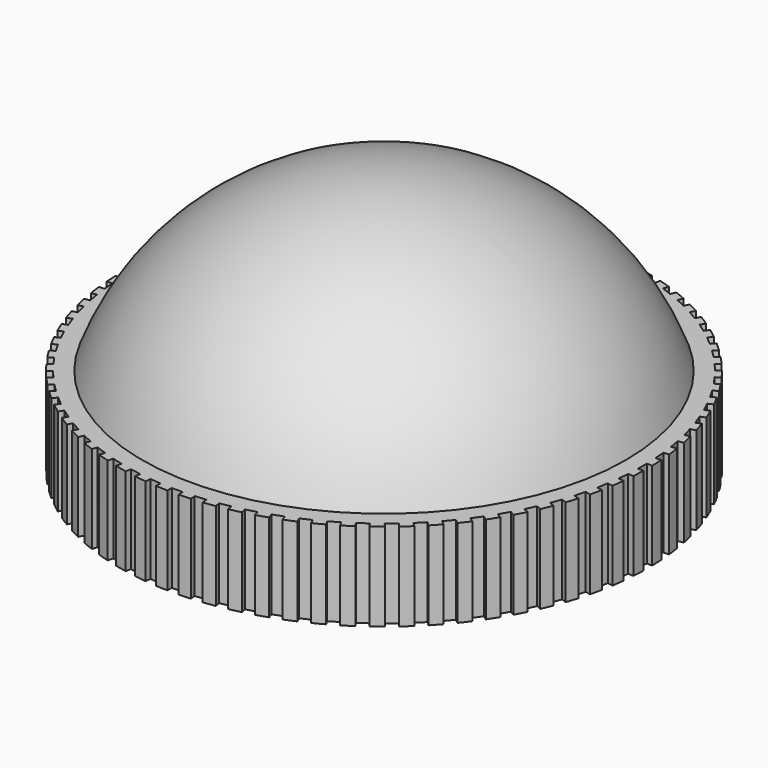
from build123d import *

# Parameters (mm, degrees)
F0_R            = 9.525
F0_R_2          = 6.35
F1_DEPTH        = 3.175
F5_DEPTH        = 25.4
F5_COPIES_COUNT = 72


# Not quite as in the source:
# - a pattern or mirror of a feature is missing from the dataset's text; its kind, count and spacing are read off the source's solid


with BuildPart() as f1:
    # F0 (on Top) → F1 (new body)
    with BuildSketch(Plane.XY):
        Circle(F0_R)
        Circle(F0_R_2, mode=Mode.SUBTRACT)
    extrude(amount=F1_DEPTH)

    # F4 (on face) → F5 (cut)
    with BuildSketch(Plane.XY.offset(3.175)):
        with BuildLine():
            Line((0.1984375, -9.5229327184), (0.1984375, -9.3265625))
            Line((0.1984375, -9.3265625), (-0.1984375, -9.3265625))
            Line((-0.1984375, -9.3265625), (-0.1984375, -9.5229327184))
            ThreePointArc((-0.1984375, -9.5229327184), (0, -9.525), (0.1984375, -9.5229327184))
        make_face()
        with BuildLine():
            Line((0.1984375, -9.7234375), (0.1984375, -9.5229327184))
            ThreePointArc((0.1984375, -9.5229327184), (0, -9.525), (-0.1984375, -9.5229327184))
            Line((-0.1984375, -9.5229327184), (-0.1984375, -9.7234375))
            Line((-0.1984375, -9.7234375), (0.1984375, -9.7234375))
        make_face()
    f5 = extrude(amount=-F5_DEPTH, mode=Mode.SUBTRACT)

    # F5_copies: F5 ×72 about axis
    f5_copies_axis = Axis((0, 0, 0), (0, 0, 1))
    for i in range(1, F5_COPIES_COUNT):
        add(f5.rotate(f5_copies_axis, i * 360 / F5_COPIES_COUNT), mode=Mode.SUBTRACT)


with BuildPart() as f3:
    # F2 (on Front) → F3 (revolve)
    with BuildSketch(Plane.XZ):
        with BuildLine():
            Line((0, 9.2906055541), (0, 1.5875))
            Line((0, 1.5875), (6.35, 1.5875))
            Line((6.35, 1.5875), (6.35, 3.175))
            Line((6.35, 3.175), (8.73125, 3.175))
            ThreePointArc((8.73125, 3.175), (5.3299943212, 7.6096328491), (0, 9.2906055541))
        make_face()
    revolve(axis=Axis((0, 0, 5.4390527771), (0, 0, -1)))


solid = Compound([f1.part, f3.part])
